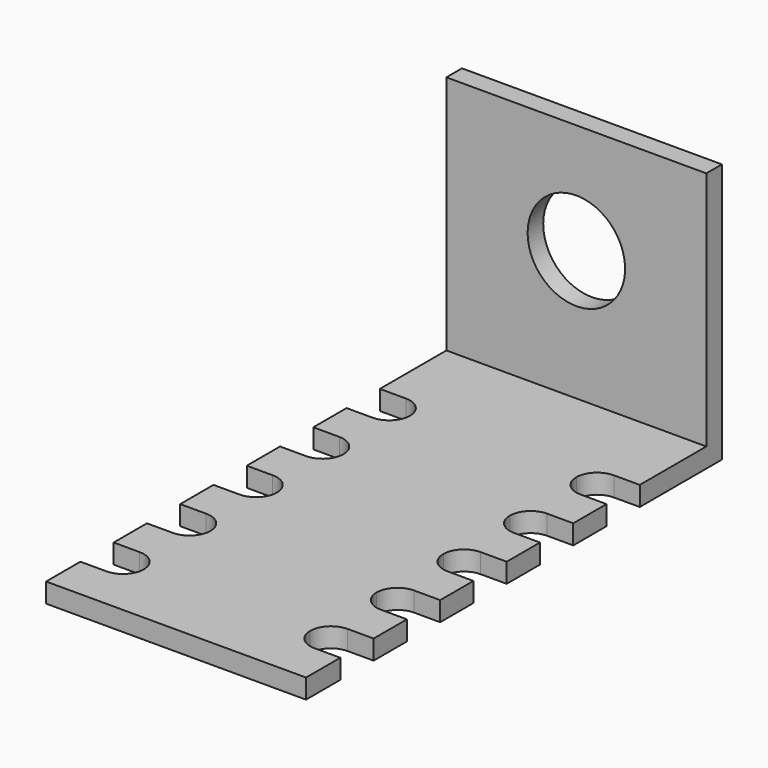
from build123d import *

# Parameters (mm, degrees)
F1_DEPTH = 1.5
F0_W     = 20
F0_H     = 1.5
F2_DEPTH = 20
F3_R     = 3.75
F4_DEPTH = 25
F5_R     = 1.59999


# Not quite as in the source:
# - a fillet or chamfer is up to 0.001 mm smaller than in the source, because OpenCascade refuses the exact size


with BuildPart() as f1:
    # F0 (on Top) → F1 (new body)
    with BuildSketch(Plane.XY):
        Polygon((0, 3.3), (0, 0), (20, 0), (20, 3.3), (16.4, 3.3), (16.4, 6.5), (20, 6.5), (20, 9.7), (16.4, 9.7), (16.4, 12.9), (20, 12.9), (20, 16.1), (16.4, 16.1), (16.4, 19.3), (20, 19.3), (20, 22.5), (16.4, 22.5), (16.4, 25.7), (20, 25.7), (20, 28.9), (16.4, 28.9), (16.4, 32.1), (20, 32.1), (20, 38.5), (0, 38.5), (0, 32.1), (3.6, 32.1), (3.6, 28.9), (0, 28.9), (0, 25.7), (3.6, 25.7), (3.6, 22.5), (0, 22.5), (0, 19.3), (3.6, 19.3), (3.6, 16.1), (0, 16.1), (0, 12.9), (3.6, 12.9), (3.6, 9.7), (0, 9.7), (0, 6.5), (3.6, 6.5), (3.6, 3.3), align=None)
    extrude(amount=F1_DEPTH)

    # F0 (on Top) → F2 (join)
    with BuildSketch(Plane.XY):
        with Locations((10, 39.25)):
            Rectangle(F0_W, F0_H)
    extrude(amount=F2_DEPTH)

    # F3 (on face) → F4 (cut)
    with BuildSketch(Plane(origin=(0, 40, 0), x_dir=(-1, 0, 0), z_dir=(0, 1, 0))):
        with Locations((-10, 11.5)):
            Circle(F3_R)
    extrude(amount=-F4_DEPTH, mode=Mode.SUBTRACT)

    # F5 (radius 1.6 in the source; OpenCascade refuses exactly that, so slightly less here)
    f5_edges = [f1.edges().sort_by_distance(p)[0] for p in [
        (16.4, 32.1, 0.75),
        (16.4, 28.9, 0.75),
        (16.4, 25.7, 0.75),
        (16.4, 22.5, 0.75),
        (16.4, 16.1, 0.75),
        (16.4, 9.7, 0.75),
        (16.4, 3.3, 0.75),
        (16.4, 19.3, 0.75),
        (16.4, 12.9, 0.75),
        (16.4, 6.5, 0.75),
        (3.6, 32.1, 0.75),
        (3.6, 25.7, 0.75),
        (3.6, 19.3, 0.75),
        (3.6, 12.9, 0.75),
        (3.6, 6.5, 0.75),
        (3.6, 28.9, 0.75),
        (3.6, 22.5, 0.75),
        (3.6, 16.1, 0.75),
        (3.6, 9.7, 0.75),
        (3.6, 3.3, 0.75),
    ]]
    fillet(f5_edges, radius=F5_R)


solid = f1.part
